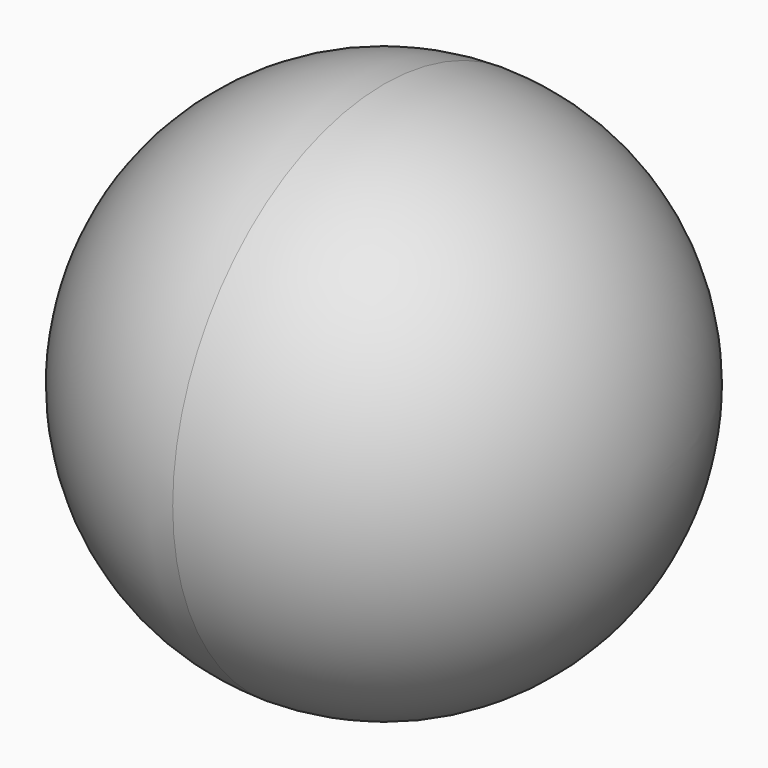
from build123d import *


# Not quite as in the source:
# - a feature of the source that left no trace in its solid (it failed there, or was rolled back) is left out


with BuildPart() as f1:
    # F0 (on Top) → F1 (revolve)
    with BuildSketch(Plane.XY):
        with BuildLine():
            Line((0, 76.2), (0, 0))
            Line((0, 0), (76.2, 0))
            ThreePointArc((76.2, 0), (53.8815367264, 53.8815367264), (0, 76.2))
        make_face()
        with BuildLine():
            Line((-76.2, 0), (0, 0))
            Line((0, 0), (0, 76.2))
            ThreePointArc((0, 76.2), (-53.8815367264, 53.8815367264), (-76.2, 0))
        make_face()
    revolve(axis=Axis((38.1, 0, 0), (1, 0, 0)))


with BuildPart() as f2:
    # F0 (on Top) → F2 (revolve)
    with BuildSketch(Plane.XY):
        with BuildLine():
            Line((0, 76.2), (0, 0))
            Line((0, 0), (76.2, 0))
            ThreePointArc((76.2, 0), (53.8815367264, 53.8815367264), (0, 76.2))
        make_face()
    revolve(axis=Axis((38.1, 0, 0), (1, 0, 0)))


solid = Compound([f1.part, f2.part])
